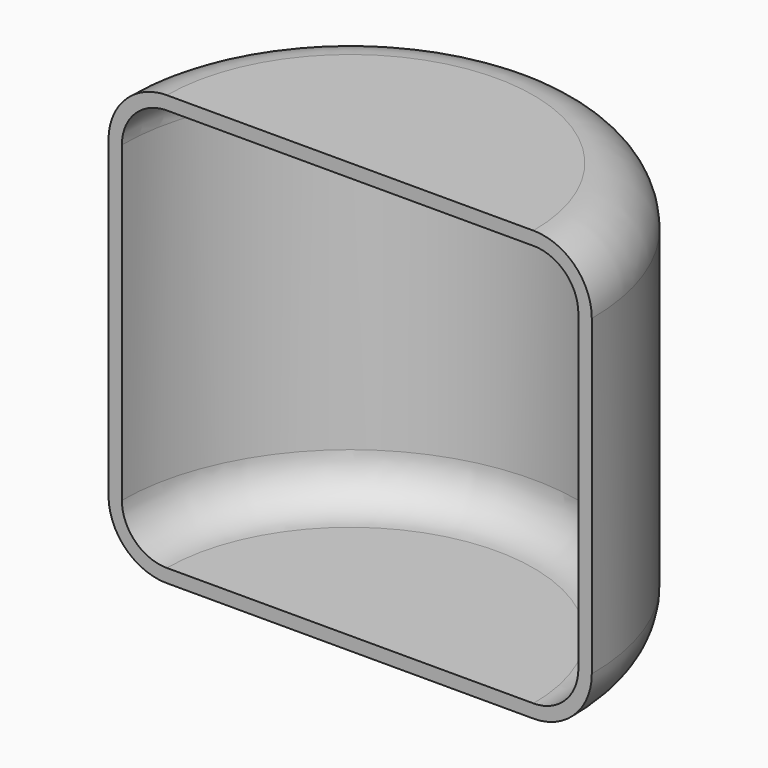
from build123d import *

# Parameters (mm, degrees)
F1_DEPTH = 406.4
F2_R     = 55.1942
F4_T     = -12.7


# Not quite as in the source:
# - two fillets or chamfers of one size are made in one step


with BuildPart() as f1:
    # F0 (on Top) → F1 (new body)
    with BuildSketch(Plane.XY):
        with BuildLine():
            ThreePointArc((228.6, 0), (0, 228.6), (-228.6, 0))
            Line((-228.6, 0), (228.6, 0))
        make_face()
    extrude(amount=F1_DEPTH)

    # F2
    f2_edges = [f1.edges().sort_by_distance(p)[0] for p in [
        (0, 228.6, 406.4),
        (0, 228.6, 0),
    ]]
    fillet(f2_edges, radius=F2_R)

    # F4
    f4_openings = [f1.faces().sort_by_distance(p)[0] for p in [
        (0, 0, 203.2),
    ]]
    offset(amount=F4_T, openings=f4_openings)


solid = f1.part
